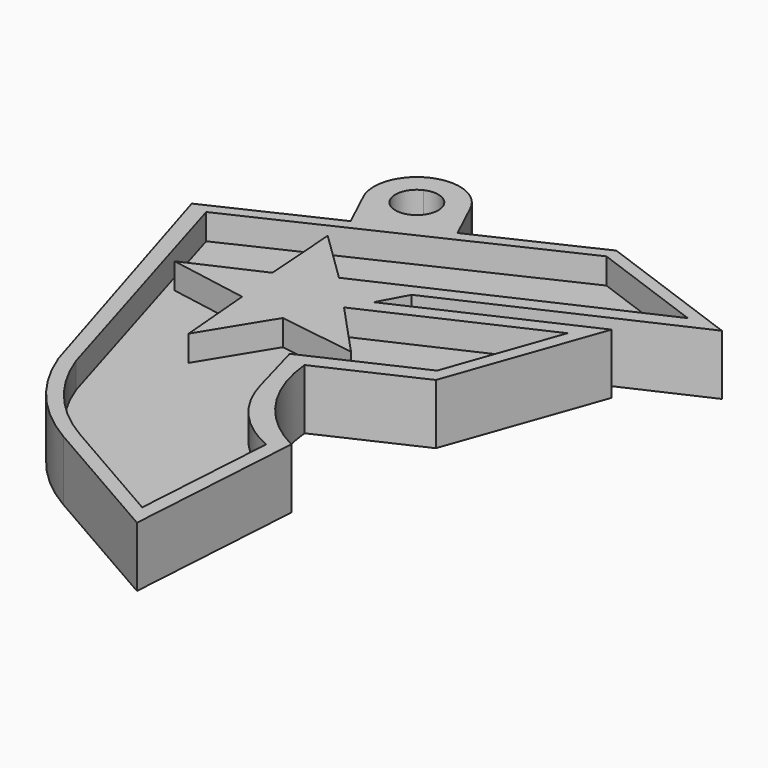
from build123d import *

# Parameters (mm, degrees)
F1_DEPTH = 7
F3_DEPTH = 4


# Not quite as in the source:
# - a feature names something its author has since deleted; it is built from what else it names


with BuildPart() as f1:
    # F0 (on Top) → F1 (new body)
    with BuildSketch(Plane.XY):
        with BuildLine():
            Line((-19.6469386943, 23.4024446265), (-33.1021886284, 17.0788295944))
            Line((-33.1021886284, 17.0788295944), (-23.5166549683, -14.3096297979))
            ThreePointArc((-23.5166549683, -14.3096297979), (-19.5683456994, -21.0463448921), (-13.5673098266, -26.0423477739))
            Line((-13.5673098266, -26.0423477739), (2.2953252774, -35.1469367743))
            Line((2.2953252774, -35.1469367743), (3.609388601, -14.3096297979))
            ThreePointArc((3.609388601, -14.3096297979), (-2.48073947, -8.9765820448), (-5.2136145532, -1.3567098649))
            Line((-5.2136145532, -1.3567098649), (5.9560768355, 3.8057526561))
            Line((5.9560768355, 3.8057526561), (12.2448138941, 21.5456220774))
            Line((12.2448138941, 21.5456220774), (-8.0293232526, 12.2533091797))
            Line((-8.0293232526, 12.2533091797), (-6.2459499526, 15.5384703992))
            Line((-6.2459499526, 15.5384703992), (20.2230613727, 27.64663617))
            Line((20.2230613727, 27.64663617), (2.8586395134, 33.9794768895))
            Line((2.8586395134, 33.9794768895), (-10.5966104207, 27.6558618574))
            Line((-10.5966104207, 27.6558618574), (-15.1217745575, 25.529153242))
            Line((-15.1217745575, 25.529153242), (-19.6469386943, 23.4024446265))
        make_face()
        with BuildLine():
            Line((-21.966829896, -13.6883575469), (-31.0345193002, 16.6006959636))
            Line((-31.0345193002, 16.6006959636), (2.8586395134, 32.5295928335))
            Line((2.8586395134, 32.5295928335), (16.2475313521, 27.64663617))
            Line((16.2475313521, 27.64663617), (-13.5077397905, 14.0351812079))
            Line((-13.5077397905, 14.0351812079), (-19.4805990905, 19.85604316))
            Line((-19.4805990905, 19.85604316), (-18.8491754234, 11.0161071643))
            Line((-18.8491754234, 11.0161071643), (-27.2155441344, 7.2275632992))
            Line((-27.2155441344, 7.2275632992), (-18.0598944426, 5.6095388718))
            Line((-18.0598944426, 5.6095388718), (-17.3100791872, -3.1120055355))
            Line((-17.3100791872, -3.1120055355), (-12.5349350274, 4.6624024399))
            Line((-12.5349350274, 4.6624024399), (-3.5371426493, 3.3206269145))
            Line((-3.5371426493, 3.3206269145), (-9.4962064177, 9.7532588989))
            Line((-9.4962064177, 9.7532588989), (9.5593021267, 18.4870336848))
            Line((9.5593021267, 18.4870336848), (4.8924595123, 5.3223588356))
            Line((4.8924595123, 5.3223588356), (-7.6506364332, -0.4748705114))
            Line((-7.6506364332, -0.4748705114), (-5.8260546066, -7.0584053174))
            ThreePointArc((-5.8260546066, -7.0584053174), (-2.996906843, -12.2802585435), (1.8299611984, -15.7404858619))
            Line((1.8299611984, -15.7404858619), (0.7740783702, -32.4837844721))
            Line((0.7740783702, -32.4837844721), (-12.6359384992, -24.7869112046))
            ThreePointArc((-12.6359384992, -24.7869112046), (-18.2844119376, -20.0640956756), (-21.966829896, -13.6883575469))
        make_face(mode=Mode.SUBTRACT)
        with BuildLine():
            Line((-21.7736473098, 27.9276087633), (-19.6469386943, 23.4024446265))
            Line((-19.6469386943, 23.4024446265), (-15.1217745575, 25.529153242))
            Line((-15.1217745575, 25.529153242), (-10.5966104207, 27.6558618574))
            Line((-10.5966104207, 27.6558618574), (-12.7233190362, 32.1810259942))
            ThreePointArc((-12.7233190362, 32.1810259942), (-15.5525190095, 34.7579017095), (-19.3751917885, 34.5794815155))
            ThreePointArc((-19.3751917885, 34.5794815155), (-21.9520675037, 31.7502815423), (-21.7736473098, 27.9276087633))
        make_face()
        with BuildLine():
            ThreePointArc((-18.3118374807, 32.3168994471), (-14.9859011046, 31.1176716865), (-16.1851288653, 27.7917353104))
            ThreePointArc((-16.1851288653, 27.7917353104), (-19.5110652414, 28.990963071), (-18.3118374807, 32.3168994471))
        make_face(mode=Mode.SUBTRACT)
    extrude(amount=F1_DEPTH)

    # F2 (on face) → F3 (join)
    with BuildSketch(Plane(origin=(0, 0, 0), x_dir=(1, 0, 0), z_dir=(0, 0, -1))):
        with BuildLine():
            ThreePointArc((-12.6359384992, 24.7869112046), (-18.2844119376, 20.0640956756), (-21.966829896, 13.6883575469))
            Line((-21.966829896, 13.6883575469), (-31.0345193002, -16.6006959636))
            Line((-31.0345193002, -16.6006959636), (2.8586395134, -32.5295928335))
            Line((2.8586395134, -32.5295928335), (16.2475313521, -27.64663617))
            Line((16.2475313521, -27.64663617), (-13.5077397905, -14.0351812079))
            Line((-13.5077397905, -14.0351812079), (-19.4805990905, -19.85604316))
            Line((-19.4805990905, -19.85604316), (-18.8491754234, -11.0161071643))
            Line((-18.8491754234, -11.0161071643), (-27.2155441344, -7.2275632992))
            Line((-27.2155441344, -7.2275632992), (-18.0598944426, -5.6095388718))
            Line((-18.0598944426, -5.6095388718), (-17.3100791872, 3.1120055355))
            Line((-17.3100791872, 3.1120055355), (-12.5349350274, -4.6624024399))
            Line((-12.5349350274, -4.6624024399), (-3.5371426493, -3.3206269145))
            Line((-3.5371426493, -3.3206269145), (-9.4962064177, -9.7532588989))
            Line((-9.4962064177, -9.7532588989), (9.5593021267, -18.4870336848))
            Line((9.5593021267, -18.4870336848), (4.8924595123, -5.3223588356))
            Line((4.8924595123, -5.3223588356), (-7.6506364332, 0.4748705114))
            Line((-7.6506364332, 0.4748705114), (-5.8260546066, 7.0584053174))
            ThreePointArc((-5.8260546066, 7.0584053174), (-2.996906843, 12.2802585435), (1.8299611984, 15.7404858619))
            Line((1.8299611984, 15.7404858619), (0.7740783702, 32.4837844721))
            Line((0.7740783702, 32.4837844721), (-12.6359384992, 24.7869112046))
        make_face()
    extrude(amount=-F3_DEPTH)


solid = f1.part
